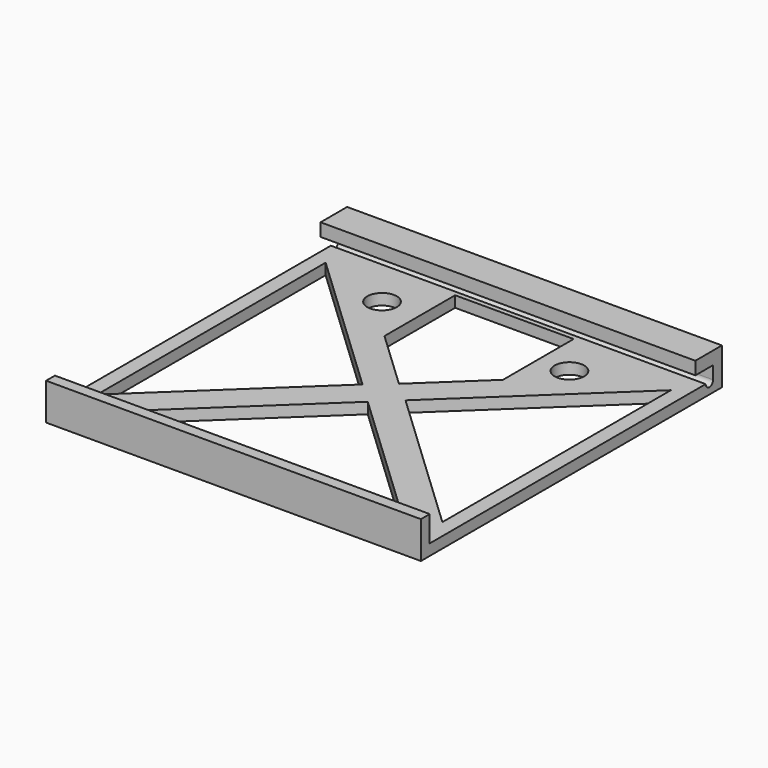
from build123d import *

# Parameters (mm, degrees)
F0_R     = 2
F1_DEPTH = 1.5
F0_W     = 50.8
F0_H     = 1.5
F2_DEPTH = 5
F3_DEPTH = 5
F4_W     = 50.8
F4_H     = 1.75
F5_DEPTH = 3
F7_DEPTH = 50.801


with BuildPart() as f1:
    # F0 (on Top) → F1 (new body)
    with BuildSketch(Plane.XY):
        Polygon((25.4, 24), (-25.4, 24), (0, 0), align=None)
        Polygon((-8.0304443836, 10.1160742342), (-8.0304443836, 22.0862291753), (8.0304443836, 22.0862291753), (8.0304443836, 10.1160742342), (0, 2.5282527694), align=None, mode=Mode.SUBTRACT)
        with Locations((-13.1485247985, 16.1011517048)):
            Circle(F0_R, mode=Mode.SUBTRACT)
        with Locations((12.2514752015, 16.1011517048)):
            Circle(F0_R, mode=Mode.SUBTRACT)
        Polygon((0, 0), (-25.4, 24), (-25.4, -24), align=None)
        Polygon((-23.3999999466, 19.3586534352), (-2.9120917277, 0), (-23.3999999466, -19.3586534352), align=None, mode=Mode.SUBTRACT)
        Polygon((0, 0), (-25.4, -24), (25.4, -24), align=None)
        Polygon((20.3712416834, -22), (-20.3712416834, -22), (0, -2.7515826614), align=None, mode=Mode.SUBTRACT)
        Polygon((25.4, -24), (25.4, 24), (0, 0), align=None)
        Polygon((23.4, -19.3586535591), (2.91209165, 0), (23.4, 19.3586535591), align=None, mode=Mode.SUBTRACT)
    extrude(amount=F1_DEPTH)

    # F0 (on Top) → F2 (join)
    with BuildSketch(Plane.XY):
        with Locations((0, -24.75)):
            Rectangle(F0_W, F0_H)
    extrude(amount=F2_DEPTH)

    # F0 (on Top) → F3 (join)
    with BuildSketch(Plane.XY):
        with Locations((0, 24.75)):
            Rectangle(F0_W, F0_H)
    extrude(amount=F3_DEPTH)

    # F4 (on face) → F5 (join)
    with BuildSketch(Plane.XZ.offset(-24)):
        with Locations((0, 4.125)):
            Rectangle(F4_W, F4_H)
    extrude(amount=F5_DEPTH)

    # F6 (on face) → F7 (cut, through all)
    with BuildSketch(Plane(origin=(-25.4, 0, 0), x_dir=(0, -1, 0), z_dir=(-1, 0, 0))):
        with BuildLine():
            ThreePointArc((-24, 1.5), (-23.375, 0.875), (-22.75, 1.5))
            Line((-22.75, 1.5), (-24, 1.5))
        make_face()
    extrude(amount=-F7_DEPTH, mode=Mode.SUBTRACT)


solid = f1.part
